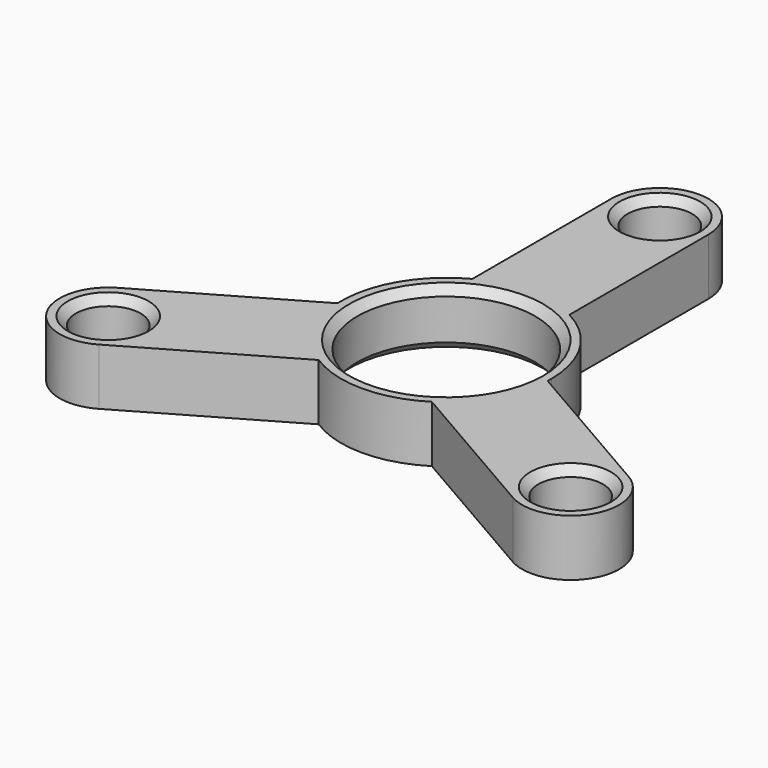
from build123d import *

# Parameters (mm, degrees)
F0_R     = 11
F0_R_2   = 4
F1_DEPTH = 3.5
F2_SIZE  = 1


# Not quite as in the source:
# - a feature names something its author has since deleted; it is built from what else it names


with BuildPart() as f1:
    # F0 (on Top) → F1 (new body, symmetric)
    with BuildSketch(Plane.XY):
        with BuildLine():
            ThreePointArc((-6, 11.5325625947), (0, 13), (6, 11.5325625947))
            Line((6, 11.5325625947), (6, 33))
            ThreePointArc((6, 33), (0, 27), (-6, 33))
            Line((-6, 33), (-6, 11.5325625947))
        make_face()
        with BuildLine():
            ThreePointArc((-6.9874921777, -10.96243372), (-11.2583302492, -6.5), (-12.9874921777, -0.5701288746))
            Line((-12.9874921777, -0.5701288746), (-31.5788383249, -11.3038475773))
            ThreePointArc((-31.5788383249, -11.3038475773), (-25.5788383249, -11.3038475773), (-22.5788383249, -16.5))
            ThreePointArc((-22.5788383249, -16.5), (-23.3826859022, -19.5), (-25.5788383249, -21.6961524227))
            Line((-25.5788383249, -21.6961524227), (-6.9874921777, -10.96243372))
        make_face()
        with BuildLine():
            Line((31.5788383249, -11.3038475773), (12.9874921777, -0.5701288746))
            ThreePointArc((12.9874921777, -0.5701288746), (11.2583302492, -6.5), (6.9874921777, -10.96243372))
            Line((6.9874921777, -10.96243372), (25.5788383249, -21.6961524227))
            ThreePointArc((25.5788383249, -21.6961524227), (23.3826859022, -13.5), (31.5788383249, -11.3038475773))
        make_face()
        with BuildLine():
            ThreePointArc((12.9874921777, -0.5701288746), (12.9968726683, -0.2851330301), (13, 0))
            ThreePointArc((13, 0), (11.1130553854, 6.7453687816), (6, 11.5325625947))
            ThreePointArc((6, 11.5325625947), (0, 13), (-6, 11.5325625947))
            ThreePointArc((-6, 11.5325625947), (-11.2583302492, 6.5), (-12.9874921777, -0.5701288746))
            ThreePointArc((-12.9874921777, -0.5701288746), (-11.2583302492, -6.5), (-6.9874921777, -10.96243372))
            ThreePointArc((-6.9874921777, -10.96243372), (0, -13), (6.9874921777, -10.96243372))
            ThreePointArc((6.9874921777, -10.96243372), (11.2583302492, -6.5), (12.9874921777, -0.5701288746))
        make_face()
        Circle(F0_R, mode=Mode.SUBTRACT)
        with BuildLine():
            ThreePointArc((-6, 33), (0, 27), (6, 33))
            ThreePointArc((6, 33), (0, 39), (-6, 33))
        make_face()
        with Locations((0, 33)):
            Circle(F0_R_2, mode=Mode.SUBTRACT)
        with BuildLine():
            ThreePointArc((-22.5788383249, -16.5), (-25.5788383249, -11.3038475773), (-31.5788383249, -11.3038475773))
            ThreePointArc((-31.5788383249, -11.3038475773), (-33.7749907476, -19.5), (-25.5788383249, -21.6961524227))
            ThreePointArc((-25.5788383249, -21.6961524227), (-23.3826859022, -19.5), (-22.5788383249, -16.5))
        make_face()
        with Locations((-28.5788383249, -16.5)):
            Circle(F0_R_2, mode=Mode.SUBTRACT)
        with BuildLine():
            ThreePointArc((34.5788383249, -16.5), (33.7749907476, -13.5), (31.5788383249, -11.3038475773))
            ThreePointArc((31.5788383249, -11.3038475773), (23.3826859022, -13.5), (25.5788383249, -21.6961524227))
            ThreePointArc((25.5788383249, -21.6961524227), (31.5788383249, -21.6961524227), (34.5788383249, -16.5))
        make_face()
        with Locations((28.5788383249, -16.5)):
            Circle(F0_R_2, mode=Mode.SUBTRACT)
    extrude(amount=F1_DEPTH, both=True)

    # F2
    f2_edges = [f1.edges().sort_by_distance(p)[0] for p in [
        (-4, 33, 3.5),
        (-11, 0, 3.5),
        (-32.578838, -16.5, 3.5),
        (24.578838, -16.5, 3.5),
        (-32.578838, -16.5, -3.5),
        (-11, 0, -3.5),
        (24.578838, -16.5, -3.5),
        (-4, 33, -3.5),
    ]]
    chamfer(f2_edges, length=F2_SIZE)


solid = f1.part
